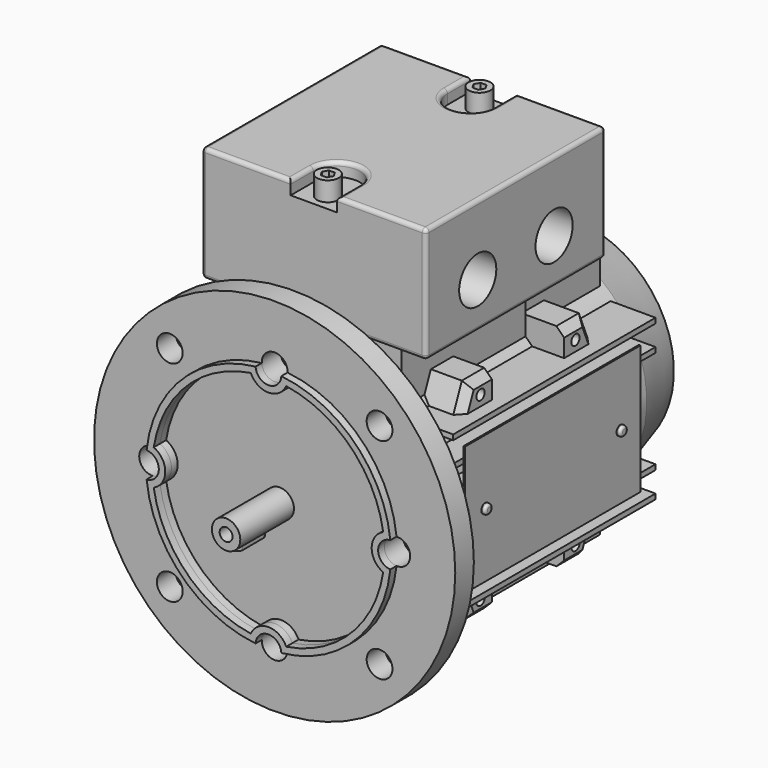
from build123d import *

# Parameters (mm, degrees)
F0_R           = 70
F1_DEPTH       = 9
F2_R           = 5
F3_DEPTH       = 9
F4_R           = 5
F5_DEPTH       = 9.001
F7_DEPTH       = 3
F9_DEPTH       = 3
F10_R          = 5.5
F11_DEPTH      = 23
F11_DEPTH_BACK = 3
F14_R          = 45
F15_DEPTH      = 115
F16_W          = 98
F16_H          = 2
F16_W_2        = 85
F17_DEPTH      = 50
F19_W          = 87
F19_H          = 87
F20_DEPTH      = 44.68
F21_W          = 12
F21_H          = 12
F22_DEPTH      = 18
F23_W          = 60
F23_H          = 60
F24_REACH      = 210.853814
F26_DEPTH      = 45
F27_SIZE       = 3
F27_2_SIZE     = 3
F27_3_SIZE     = 3
F27_4_SIZE     = 3
F28_R          = 2
F29_DEPTH      = 10
F30_R          = 2
F31_DEPTH      = 10
F32_R          = 2
F33_DEPTH      = 9
F34_W          = 85
F34_H          = 50
F35_DEPTH      = 0.6
F36_R          = 1.875
F37_DEPTH      = 1.5
F38_R          = 1
F40_DEPTH      = 5.25
F41_R          = 4.25
F42_DEPTH      = 7.5
F44_DEPTH      = 4
F45_R          = 1.5
F46_R          = 1
F46_2_R        = 1
F46_3_R        = 1
F46_4_R        = 1
F47_R          = 9
F48_DEPTH      = 12
F49_R          = 45
F51_R          = 39
F53_R          = 1
F54_R          = 5.5
F55_DEPTH      = 22
F57_DEPTH      = 22
F59_DEPTH      = 7
F60_R          = 2.5
F61_DEPTH      = 15
F62_W          = 2
F62_H          = 98
F62_H_2        = 85
F63_DEPTH      = 50
F64_W          = 2
F64_H          = 38
F64_H_2        = 30
F65_DEPTH      = 50


# Not quite as in the source:
# - after a boolean that leaves OpenCascade's solid faulty, fix() repairs it


with BuildPart() as f1:
    # F0 (on Front) → F1 (new body)
    with BuildSketch(Plane.XZ):
        Circle(F0_R)
    extrude(amount=-F1_DEPTH)

    # F2 (on face) → F3 (cut, through all)
    with BuildSketch(Plane.XZ):
        with Locations((-40.65864, 40.65864)):
            Circle(F2_R)
        with Locations((-40.65864, -40.65864)):
            Circle(F2_R)
        with Locations((40.65864, -40.65864)):
            Circle(F2_R)
        with Locations((40.65864, 40.65864)):
            Circle(F2_R)
    extrude(amount=-F3_DEPTH, mode=Mode.SUBTRACT)

    # F4 (on face) → F5 (cut, through all)
    with BuildSketch(Plane.XZ):
        with Locations((0, 47.5)):
            Circle(F4_R)
        with Locations((47.5, 0)):
            Circle(F4_R)
        with Locations((0, -47.5)):
            Circle(F4_R)
        with Locations((-47.5, 0)):
            Circle(F4_R)
    extrude(amount=-F5_DEPTH, mode=Mode.SUBTRACT)

    # F6 (on Front) → F7 (join)
    with BuildSketch(Plane.XZ):
        with BuildLine():
            ThreePointArc((4.99307, 47.236842), (0, 42.5), (-4.99307, 47.236842))
            ThreePointArc((-4.99307, 47.236842), (-33.587572, 33.587572), (-47.236842, 4.99307))
            ThreePointArc((-47.236842, 4.99307), (-42.5, 0), (-47.236842, -4.99307))
            ThreePointArc((-47.236842, -4.99307), (-33.587572, -33.587572), (-4.99307, -47.236842))
            ThreePointArc((-4.99307, -47.236842), (0, -42.5), (4.99307, -47.236842))
            ThreePointArc((4.99307, -47.236842), (33.587572, -33.587572), (47.236842, -4.99307))
            ThreePointArc((47.236842, -4.99307), (42.5, 0), (47.236842, 4.99307))
            ThreePointArc((47.236842, 4.99307), (33.587572, 33.587572), (4.99307, 47.236842))
        make_face()
        with BuildLine():
            ThreePointArc((44.473684, -6.862318), (31.819805, -31.819805), (6.862318, -44.473684))
            ThreePointArc((6.862318, -44.473684), (0, -40), (-6.862318, -44.473684))
            ThreePointArc((-6.862318, -44.473684), (-31.819805, -31.819805), (-44.473684, -6.862318))
            ThreePointArc((-44.473684, -6.862318), (-40, 0), (-44.473684, 6.862318))
            ThreePointArc((-44.473684, 6.862318), (-31.819805, 31.819805), (-6.862318, 44.473684))
            ThreePointArc((-6.862318, 44.473684), (0, 40), (6.862318, 44.473684))
            ThreePointArc((6.862318, 44.473684), (31.819805, 31.819805), (44.473684, 6.862318))
            ThreePointArc((44.473684, 6.862318), (40, 0), (44.473684, -6.862318))
        make_face(mode=Mode.SUBTRACT)
    extrude(amount=F7_DEPTH)

    add(f1.part.fix(), mode=Mode.REPLACE)

    # F8 (on face) → F9 (cut)
    with BuildSketch(Plane.XZ):
        with BuildLine():
            ThreePointArc((6.862318, 44.473684), (0, 40), (-6.862318, 44.473684))
            ThreePointArc((-6.862318, 44.473684), (-31.819805, 31.819805), (-44.473684, 6.862318))
            ThreePointArc((-44.473684, 6.862318), (-40, 0), (-44.473684, -6.862318))
            ThreePointArc((-44.473684, -6.862318), (-31.819805, -31.819805), (-6.862318, -44.473684))
            ThreePointArc((-6.862318, -44.473684), (0, -40), (6.862318, -44.473684))
            ThreePointArc((6.862318, -44.473684), (31.819805, -31.819805), (44.473684, -6.862318))
            ThreePointArc((44.473684, -6.862318), (40, 0), (44.473684, 6.862318))
            ThreePointArc((44.473684, 6.862318), (31.819805, 31.819805), (6.862318, 44.473684))
        make_face()
    extrude(amount=-F9_DEPTH, mode=Mode.SUBTRACT)


with BuildPart() as f11:
    # F10 (on face) → F11 (new body, two sides)
    with BuildSketch(Plane.XZ) as f11_sk:
        with Locations((-0.429371, -0.420938)):
            Circle(F10_R)
    extrude(amount=F11_DEPTH)
    extrude(f11_sk.sketch, amount=-F11_DEPTH_BACK)

    # F58 (on Top) → F59 (join)
    with BuildSketch(Plane.XY):
        with BuildLine():
            Line((-2, -8), (-2, -18))
            ThreePointArc((-2, -18), (-1.414214, -19.414214), (0, -20))
            ThreePointArc((0, -20), (1.414214, -19.414214), (2, -18))
            Line((2, -18), (2, -8))
            ThreePointArc((2, -8), (1.414214, -6.585786), (0, -6))
            ThreePointArc((0, -6), (-1.414214, -6.585786), (-2, -8))
        make_face()
    extrude(amount=-F59_DEPTH)

    # F60 (on face) → F61 (cut)
    with BuildSketch(Plane.XZ.offset(23)):
        with Locations((-0.429371, -0.420938)):
            Circle(F60_R)
    extrude(amount=-F61_DEPTH, mode=Mode.SUBTRACT)


with BuildPart() as f15:
    # F14 (on face) → F15 (new body)
    with BuildSketch(Plane(origin=(0, 9, 0), x_dir=(-1, 0, 0), z_dir=(0, 1, 0))):
        Circle(F14_R)
    extrude(amount=F15_DEPTH)

    # F16 (on Right) → F17 (join, symmetric)
    with BuildSketch(Plane.YZ):
        with Locations((73, 20)):
            Rectangle(F16_W, F16_H)
        with Locations((71.5, 10)):
            Rectangle(F16_W_2, F16_H)
        with Locations((71.5, 0)):
            Rectangle(F16_W_2, F16_H)
        with Locations((73, 30)):
            Rectangle(F16_W, F16_H)
        with Locations((71.5, -10)):
            Rectangle(F16_W_2, F16_H)
        with Locations((73, -20)):
            Rectangle(F16_W, F16_H)
        with Locations((73, -30)):
            Rectangle(F16_W, F16_H)
    extrude(amount=F17_DEPTH, both=True)


with BuildPart() as f20:
    # F19 (on offset) → F20 (new body)
    with BuildSketch(Plane.XY.offset(56)):
        with Locations((0, 62.5)):
            Rectangle(F19_W, F19_H)
    extrude(amount=F20_DEPTH)

    # F39 (on face) → F40 (cut)
    with BuildSketch(Plane.XY.offset(100.68)):
        with BuildLine():
            Line((-9, 30), (-9, 19))
            Line((-9, 19), (0, 19))
            Line((0, 19), (9, 19))
            Line((9, 19), (9, 30))
            ThreePointArc((9, 30), (0, 39), (-9, 30))
        make_face()
        with BuildLine():
            ThreePointArc((-9, 95), (0, 86), (9, 95))
            Line((9, 95), (9, 106))
            Line((9, 106), (-9, 106))
            Line((-9, 106), (-9, 95))
        make_face()
    extrude(amount=-F40_DEPTH, mode=Mode.SUBTRACT)

    # F41 (on face) → F42 (join)
    with BuildSketch(Plane.XY.offset(95.43)):
        with Locations((0, 25.75)):
            Circle(F41_R)
        with Locations((0, 99.25)):
            Circle(F41_R)
    extrude(amount=F42_DEPTH)

    # F43 (on face) → F44 (cut)
    with BuildSketch(Plane.XY.offset(102.93)):
        Polygon((1.154701, 27.75), (-1.154701, 27.75), (-2.309401, 25.75), (-1.154701, 23.75), (1.154701, 23.75), (2.309401, 25.75), align=None)
        Polygon((1.154701, 97.25), (2.309401, 99.25), (1.154701, 101.25), (-1.154701, 101.25), (-2.309401, 99.25), (-1.154701, 97.25), align=None)
    extrude(amount=-F44_DEPTH, mode=Mode.SUBTRACT)

    # F45
    f45_edges = [f20.edges().sort_by_distance(p)[0] for p in [
        (-43.5, 62.5, 100.68),
        (-26.25, 19, 100.68),
        (-9, 24.5, 100.68),
        (0, 39, 100.68),
        (9, 24.5, 100.68),
        (26.25, 19, 100.68),
        (43.5, 62.5, 100.68),
        (26.25, 106, 100.68),
        (9, 100.5, 100.68),
        (0, 86, 100.68),
        (-9, 100.5, 100.68),
        (-26.25, 106, 100.68),
        (43.5, 19, 78.34),
        (-43.5, 19, 78.34),
        (43.5, 106, 78.34),
        (-43.5, 62.5, 56),
        (-43.5, 106, 78.34),
        (0, 106, 56),
        (43.5, 62.5, 56),
        (0, 19, 56),
    ]]
    fillet(f45_edges, radius=F45_R)

    # F47 (on face) → F48 (cut)
    with BuildSketch(Plane.YZ.offset(43.5)):
        with Locations((44, 73.5)):
            Circle(F47_R)
        with Locations((81, 73.5)):
            Circle(F47_R)
    extrude(amount=-F48_DEPTH, mode=Mode.SUBTRACT)


with BuildPart() as f22:
    # F21 (on face) → F22 (new body)
    with BuildSketch(Plane(origin=(0, 9, 0), x_dir=(-1, 0, 0), z_dir=(0, 1, 0))):
        with Locations((47.5, 0)):
            Rectangle(F21_W, F21_H)
    extrude(amount=F22_DEPTH)

    # F46#3
    f46_3_edges = [f22.edges().sort_by_distance(p)[0] for p in [
        (-53.5, 18, -6),
        (-53.5, 18, 6),
    ]]
    fillet(f46_3_edges, radius=F46_3_R)


with BuildPart() as f22b:
    # F21 (on face) → F22, piece 2 (new body)
    with BuildSketch(Plane(origin=(0, 9, 0), x_dir=(-1, 0, 0), z_dir=(0, 1, 0))):
        with Locations((0, -47.5)):
            Rectangle(F21_W, F21_H)
    extrude(amount=F22_DEPTH)

    # F46#2
    f46_2_edges = [f22b.edges().sort_by_distance(p)[0] for p in [
        (6, 18, -53.5),
        (-6, 18, -53.5),
    ]]
    fillet(f46_2_edges, radius=F46_2_R)


with BuildPart() as f22c:
    # F21 (on face) → F22, piece 3 (new body)
    with BuildSketch(Plane(origin=(0, 9, 0), x_dir=(-1, 0, 0), z_dir=(0, 1, 0))):
        with Locations((-47.5, 0)):
            Rectangle(F21_W, F21_H)
    extrude(amount=F22_DEPTH)

    # F46
    f46_edges = [f22c.edges().sort_by_distance(p)[0] for p in [
        (53.5, 18, 6),
        (53.5, 18, -6),
    ]]
    fillet(f46_edges, radius=F46_R)


with BuildPart() as f22d:
    # F21 (on face) → F22, piece 4 (new body)
    with BuildSketch(Plane(origin=(0, 9, 0), x_dir=(-1, 0, 0), z_dir=(0, 1, 0))):
        with Locations((0, 47.5)):
            Rectangle(F21_W, F21_H)
    extrude(amount=F22_DEPTH)

    # F46#4
    f46_4_edges = [f22d.edges().sort_by_distance(p)[0] for p in [
        (6, 18, 53.5),
        (-6, 18, 53.5),
    ]]
    fillet(f46_4_edges, radius=F46_4_R)


with BuildPart() as f24:
    f24_end = f15.part.faces().sort_by_distance((45, 10.715372, 0))[0]
    # F23 (on face) → F24 (new body, up to a face of F15 that its end follows)
    with BuildSketch(Plane(origin=(0, 0, 56), x_dir=(1, 0, 0), z_dir=(0, 0, -1))):
        with Locations((0, -54)):
            Rectangle(F23_W, F23_H)
    f24_long = extrude(amount=F24_REACH, mode=Mode.PRIVATE)
    add(split(f24_long, bisect_by=f24_end, keep=Keep.ALL, mode=Mode.PRIVATE).solids().sort_by_distance((0, 54, 56))[0])


with BuildPart() as f26:
    # F25 (on Right) → F26 (new body, symmetric)
    with BuildSketch(Plane.YZ):
        Polygon((34, -31), (38.166667, -41), (49, -41), (49, -31), align=None)
    extrude(amount=F26_DEPTH, both=True)

    # F27
    f27_edges = [f26.edges().sort_by_distance(p)[0] for p in [
        (45, 43.583333, -41),
        (45, 36.083333, -36),
        (-45, 43.583333, -41),
        (-45, 36.083333, -36),
    ]]
    chamfer(f27_edges, length=F27_SIZE)


with BuildPart() as f26b:
    # F25 (on Right) → F26, piece 2 (new body, symmetric)
    with BuildSketch(Plane.YZ):
        Polygon((84, -31), (84, -41), (94.833333, -41), (99, -31), align=None)
    extrude(amount=F26_DEPTH, both=True)

    # F27#2
    f27_2_edges = [f26b.edges().sort_by_distance(p)[0] for p in [
        (45, 89.416667, -41),
        (45, 96.916667, -36),
        (-45, 96.916667, -36),
        (-45, 89.416667, -41),
    ]]
    chamfer(f27_2_edges, length=F27_2_SIZE)


with BuildPart() as f26c:
    # F25 (on Right) → F26, piece 3 (new body, symmetric)
    with BuildSketch(Plane.YZ):
        Polygon((49, 41), (38.166667, 41), (34, 31), (49, 31), align=None)
    extrude(amount=F26_DEPTH, both=True)

    # F27#4
    f27_4_edges = [f26c.edges().sort_by_distance(p)[0] for p in [
        (45, 43.583333, 41),
        (45, 36.083333, 36),
        (-45, 43.583333, 41),
        (-45, 36.083333, 36),
    ]]
    chamfer(f27_4_edges, length=F27_4_SIZE)


with BuildPart() as f26d:
    # F25 (on Right) → F26, piece 4 (new body, symmetric)
    with BuildSketch(Plane.YZ):
        Polygon((94.833333, 41), (84, 41), (84, 31), (99, 31), align=None)
    extrude(amount=F26_DEPTH, both=True)

    # F27#3
    f27_3_edges = [f26d.edges().sort_by_distance(p)[0] for p in [
        (45, 96.916667, 36),
        (45, 89.416667, 41),
        (-45, 96.916667, 36),
        (-45, 89.416667, 41),
    ]]
    chamfer(f27_3_edges, length=F27_3_SIZE)


with BuildPart() as f29_tool:
    # F28 (on face) → F29 (new body)
    with BuildSketch(Plane(origin=(-45, 0, 0), x_dir=(0, -1, 0), z_dir=(-1, 0, 0))):
        with Locations((-89.5, 35)):
            Circle(F28_R)
        with Locations((-43.5, 35)):
            Circle(F28_R)
        with Locations((-89.5, -35)):
            Circle(F28_R)
        with Locations((-43.5, -35)):
            Circle(F28_R)
    extrude(amount=-F29_DEPTH)


with BuildPart() as f26_1:
    add(f26.part)

    # F29: cut by f29_tool
    add(f29_tool.part, mode=Mode.SUBTRACT)


with BuildPart() as f26b_1:
    add(f26b.part)

    # F29: cut by f29_tool
    add(f29_tool.part, mode=Mode.SUBTRACT)


with BuildPart() as f26c_1:
    add(f26c.part)

    # F29: cut by f29_tool
    add(f29_tool.part, mode=Mode.SUBTRACT)


with BuildPart() as f26d_1:
    add(f26d.part)

    # F29: cut by f29_tool
    add(f29_tool.part, mode=Mode.SUBTRACT)


with BuildPart() as f31_tool:
    # F30 (on face) → F31 (new body)
    with BuildSketch(Plane.YZ.offset(45)):
        with Locations((43.5, 35)):
            Circle(F30_R)
        with Locations((89.5, 35)):
            Circle(F30_R)
        with Locations((89.5, -35)):
            Circle(F30_R)
        with Locations((43.5, -35)):
            Circle(F30_R)
    extrude(amount=-F31_DEPTH)


with BuildPart() as f26_2:
    add(f26_1.part)

    # F31: cut by f31_tool
    add(f31_tool.part, mode=Mode.SUBTRACT)


with BuildPart() as f26b_2:
    add(f26b_1.part)

    # F31: cut by f31_tool
    add(f31_tool.part, mode=Mode.SUBTRACT)


with BuildPart() as f26c_2:
    add(f26c_1.part)

    # F31: cut by f31_tool
    add(f31_tool.part, mode=Mode.SUBTRACT)


with BuildPart() as f26d_2:
    add(f26d_1.part)

    # F31: cut by f31_tool
    add(f31_tool.part, mode=Mode.SUBTRACT)


with BuildPart() as f33_tool:
    # F32 (on face) → F33 (new body)
    with BuildSketch(Plane(origin=(0, 0, -41), x_dir=(1, 0, 0), z_dir=(0, 0, -1))):
        with Locations((35, -89.5)):
            Circle(F32_R)
        with Locations((-35, -89.5)):
            Circle(F32_R)
        with Locations((35, -43.5)):
            Circle(F32_R)
        with Locations((-35, -43.5)):
            Circle(F32_R)
    extrude(amount=-F33_DEPTH)


with BuildPart() as f26_3:
    add(f26_2.part)

    # F33: cut by f33_tool
    add(f33_tool.part, mode=Mode.SUBTRACT)


with BuildPart() as f26b_3:
    add(f26b_2.part)

    # F33: cut by f33_tool
    add(f33_tool.part, mode=Mode.SUBTRACT)


with BuildPart() as f15_1:
    add(f15.part)

    # F34 (on face) → F35 (join)
    with BuildSketch(Plane.YZ.offset(50)):
        with Locations((71.5, 0)):
            Rectangle(F34_W, F34_H)
    extrude(amount=F35_DEPTH)

    # F36 (on face) → F37 (join)
    with BuildSketch(Plane.YZ.offset(50.6)):
        with Locations((38.75, 0)):
            Circle(F36_R)
        with Locations((104.25, 0)):
            Circle(F36_R)
    extrude(amount=F37_DEPTH)

    # F38
    f38_edges = [f15_1.edges().sort_by_distance(p)[0] for p in [
        (52.1, 102.375, 0),
        (52.1, 36.875, 0),
    ]]
    fillet(f38_edges, radius=F38_R)

    # F49 (on face) → F52 section 0
    with BuildSketch(Plane(origin=(0, 124, 0), x_dir=(-1, 0, 0), z_dir=(0, 1, 0))):
        Circle(F49_R)
    # F51 (on offset) → F52 section 1
    with BuildSketch(Plane(origin=(0, 145, 0), x_dir=(-1, 0, 0), z_dir=(0, 1, 0))):
        Circle(F51_R)
    loft()

    # F53
    f53_edges = [f15_1.edges().sort_by_distance(p)[0] for p in [
        (39, 145, 0),
    ]]
    fillet(f53_edges, radius=F53_R)

    # F54 (on face) → F55 (join)
    with BuildSketch(Plane(origin=(0, 145, 0), x_dir=(-1, 0, 0), z_dir=(0, 1, 0))):
        Circle(F54_R)
    extrude(amount=F55_DEPTH)

    # F56 (on face) → F57 (cut, through all)
    with BuildSketch(Plane(origin=(0, 167, 0), x_dir=(-1, 0, 0), z_dir=(0, 1, 0))):
        Polygon((0, -3.5), (-1.9, -3.5), (-1.9, -5.5), (1.9, -5.5), (1.9, -3.5), align=None)
    extrude(amount=-F57_DEPTH, mode=Mode.SUBTRACT)

    add(f26_3.part)  # F63 merges F26

    add(f26b_3.part)  # F63 merges F26b
    # F62 (on Top) → F63 (join)
    with BuildSketch(Plane.XY):
        with Locations((-17.5, 73)):
            Rectangle(F62_W, F62_H)
        with Locations((-7.5, 71.5)):
            Rectangle(F62_W, F62_H_2)
        with Locations((0, 71.5)):
            Rectangle(F62_W, F62_H_2)
        with Locations((-27.5, 73)):
            Rectangle(F62_W, F62_H)
        with Locations((7.5, 71.5)):
            Rectangle(F62_W, F62_H_2)
        with Locations((17.5, 73)):
            Rectangle(F62_W, F62_H)
        with Locations((27.5, 73)):
            Rectangle(F62_W, F62_H)
    extrude(amount=-F63_DEPTH)

    add(f24.part)  # F65 merges F24

    add(f26d_2.part)  # F65 merges F26d
    # F64 (on Top) → F65 (join)
    with BuildSketch(Plane.XY):
        with Locations((-27.5, 103)):
            Rectangle(F64_W, F64_H)
        with Locations((-17.5, 103)):
            Rectangle(F64_W, F64_H)
        with Locations((-7.5, 99)):
            Rectangle(F64_W, F64_H_2)
        with Locations((0, 99)):
            Rectangle(F64_W, F64_H_2)
        with Locations((7.5, 99)):
            Rectangle(F64_W, F64_H_2)
        with Locations((17.5, 103)):
            Rectangle(F64_W, F64_H)
        with Locations((27.5, 103)):
            Rectangle(F64_W, F64_H)
    extrude(amount=F65_DEPTH)


solid = Compound([f1.part, f11.part, f20.part, f22.part, f22b.part, f22c.part, f22d.part, f26c_2.part, f15_1.part])
